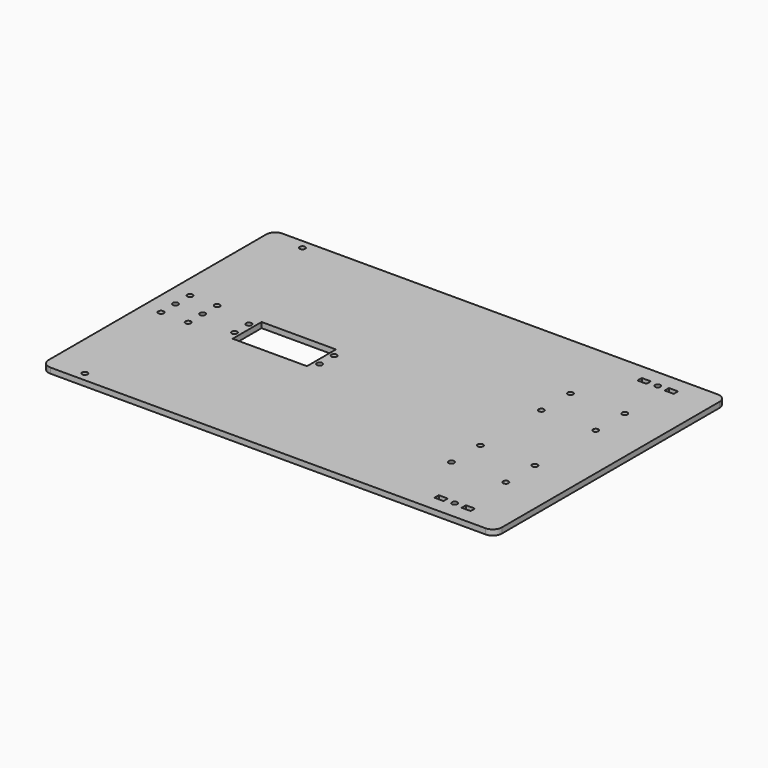
from build123d import *

# Parameters (mm, degrees)
F0_R     = 1.5
F0_W     = 5
F0_H     = 3
F0_W_2   = 41
F0_H_2   = 20
F1_DEPTH = 3


with BuildPart() as f1:
    # F0 (on Top) → F1 (new body)
    with BuildSketch(Plane.XY):
        with BuildLine():
            Line((245, 160), (5, 160))
            ThreePointArc((5, 160), (1.4644660941, 158.5355339059), (0, 155))
            Line((0, 155), (0, 5))
            ThreePointArc((0, 5), (1.4644660941, 1.4644660941), (5, 0))
            Line((5, 0), (245, 0))
            ThreePointArc((245, 0), (248.5355339059, 1.4644660941), (250, 5))
            Line((250, 5), (250, 155))
            ThreePointArc((250, 155), (248.5355339059, 158.5355339059), (245, 160))
        make_face()
        with Locations((20, 5)):
            Circle(F0_R, mode=Mode.SUBTRACT)
        with Locations((212.5, 10)):
            Rectangle(F0_W, F0_H, mode=Mode.SUBTRACT)
        with Locations((220, 10)):
            Circle(F0_R, mode=Mode.SUBTRACT)
        with Locations((227.5, 10)):
            Rectangle(F0_W, F0_H, mode=Mode.SUBTRACT)
        with Locations((195, 39)):
            Circle(F0_R, mode=Mode.SUBTRACT)
        with Locations((225, 39)):
            Circle(F0_R, mode=Mode.SUBTRACT)
        with Locations((9.9999278665, 70)):
            Circle(F0_R, mode=Mode.SUBTRACT)
        with Locations((24.9999278665, 70)):
            Circle(F0_R, mode=Mode.SUBTRACT)
        with Locations((9.9999278665, 80)):
            Circle(F0_R, mode=Mode.SUBTRACT)
        with Locations((24.9999278665, 80)):
            Circle(F0_R, mode=Mode.SUBTRACT)
        with Locations((9.9999278665, 90)):
            Circle(F0_R, mode=Mode.SUBTRACT)
        with Locations((24.9999278665, 90)):
            Circle(F0_R, mode=Mode.SUBTRACT)
        with Locations((46.5, 75)):
            Circle(F0_R, mode=Mode.SUBTRACT)
        with Locations((46.5, 85)):
            Circle(F0_R, mode=Mode.SUBTRACT)
        with Locations((70, 80)):
            Rectangle(F0_W_2, F0_H_2, mode=Mode.SUBTRACT)
        with Locations((93.5, 75)):
            Circle(F0_R, mode=Mode.SUBTRACT)
        with Locations((93.5, 85)):
            Circle(F0_R, mode=Mode.SUBTRACT)
        with Locations((20, 155)):
            Circle(F0_R, mode=Mode.SUBTRACT)
        with Locations((195, 59)):
            Circle(F0_R, mode=Mode.SUBTRACT)
        with Locations((225, 59)):
            Circle(F0_R, mode=Mode.SUBTRACT)
        with Locations((195, 101)):
            Circle(F0_R, mode=Mode.SUBTRACT)
        with Locations((195, 121)):
            Circle(F0_R, mode=Mode.SUBTRACT)
        with Locations((225, 101)):
            Circle(F0_R, mode=Mode.SUBTRACT)
        with Locations((225, 121)):
            Circle(F0_R, mode=Mode.SUBTRACT)
        with Locations((212.5, 150)):
            Rectangle(F0_W, F0_H, mode=Mode.SUBTRACT)
        with Locations((220, 150)):
            Circle(F0_R, mode=Mode.SUBTRACT)
        with Locations((227.5, 150)):
            Rectangle(F0_W, F0_H, mode=Mode.SUBTRACT)
    extrude(amount=F1_DEPTH)


solid = f1.part
